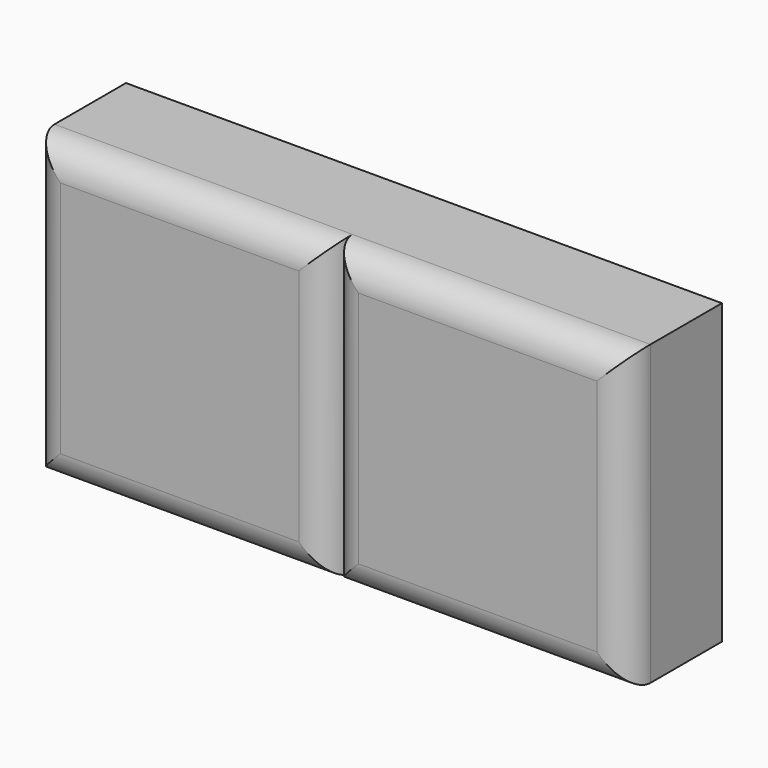
from build123d import *

# Parameters (mm, degrees)
F0_W     = 50.8
F0_H     = 50.8
F1_DEPTH = 25.4
F3_R     = 5.08
F4_SIZE  = 5.08
F5_T     = -2.54


# Not quite as in the source:
# - a feature of the source that left no trace in its solid (it failed there, or was rolled back) is left out


with BuildPart() as f1:
    # F0 (on Front) → F1 (new body)
    with BuildSketch(Plane.XZ):
        Rectangle(F0_W, F0_H)
    extrude(amount=F1_DEPTH)

    # F3
    f3_edges = [f1.edges().sort_by_distance(p)[0] for p in [
        (0, -25.4, 25.4),
        (-25.4, -25.4, 0),
        (0, -25.4, -25.4),
        (25.4, -25.4, 0),
    ]]
    fillet(f3_edges, radius=F3_R)

    # F4
    f4_edges = [f1.edges().sort_by_distance(p)[0] for p in [
        (0, 0, 25.4),
        (-25.4, 0, 0),
        (0, 0, -25.4),
        (25.4, 0, 0),
    ]]
    chamfer(f4_edges, length=F4_SIZE)

    # F5
    f5_openings = [f1.faces().sort_by_distance(p)[0] for p in [
        (0, 0, 0),
    ]]
    offset(amount=F5_T, openings=f5_openings)

    # F6: F1 across face


with BuildPart() as f1_1:
    add(f1.part)
    add(f1.part.mirror(Plane(origin=(25.4, -12.7, 0), x_dir=(0, 1, 0), z_dir=(1, 0, 0))))


solid = f1_1.part
